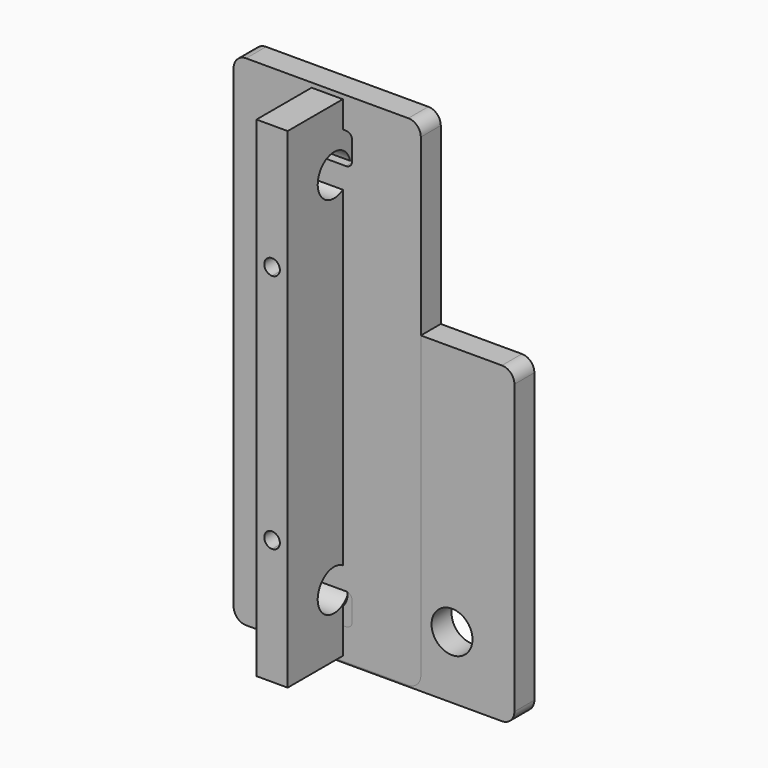
from build123d import *

# Parameters (mm, degrees)
F1_DEPTH  = 5.08
F2_R      = 2.54
F3_R      = 3.571875
F4_DEPTH  = 5.08
F5_R      = 2.54
F6_R      = 1.27
F8_DEPTH  = 19.1135
F9_R      = 4.1656
F10_DEPTH = 25.4


# Not quite as in the source:
# - a feature names something its author has since deleted; it is built from what else it names


with BuildPart() as f1:
    # F0 (on Front) → F1 (new body)
    with BuildSketch(Plane.XZ):
        with BuildLine():
            Line((-4.1654060763, -38.3941942743), (-12.7, -38.3941942743))
            Line((-12.7, -38.3941942743), (-12.7, -51.054))
            Line((-12.7, -51.054), (0, -51.054))
            Line((0, -51.054), (0, -42.5196))
            ThreePointArc((0, -42.5196), (-2.931278739, -41.3137007137), (-4.1654060763, -38.3941942743))
        make_face()
        with BuildLine():
            Line((0, -10.668), (0, -7.9375))
            ThreePointArc((0, -7.9375), (-5.6126600757, -5.6126600757), (-7.9375, 0))
            Line((-7.9375, 0), (-12.7, 0))
            Line((-12.7, 0), (-12.7, -38.3941942743))
            Line((-12.7, -38.3941942743), (-4.1654060763, -38.3941942743))
            ThreePointArc((-4.1654060763, -38.3941942743), (-2.9597007137, -35.422721261), (0, -34.1884))
            Line((0, -34.1884), (0, -10.668))
        make_face()
        with BuildLine():
            ThreePointArc((-7.9375, 0), (-5.6126600757, 5.6126600757), (0, 7.9375))
            Line((0, 7.9375), (0, 12.7))
            Line((0, 12.7), (-12.7, 12.7))
            Line((-12.7, 12.7), (-12.7, 0))
            Line((-12.7, 0), (-7.9375, 0))
        make_face()
        with BuildLine():
            ThreePointArc((0, 7.9375), (5.6126600757, 5.6126600757), (7.9375, 0))
            Line((7.9375, 0), (19.05, 0))
            Line((19.05, 0), (38.1, 0))
            Line((38.1, 0), (38.1, 12.7))
            Line((38.1, 12.7), (0, 12.7))
            Line((0, 12.7), (0, 7.9375))
        make_face()
        with BuildLine():
            Line((38.1, 0), (19.05, 0))
            Line((19.05, 0), (19.05, -38.354))
            Line((19.05, -38.354), (21.2344, -38.354))
            ThreePointArc((21.2344, -38.354), (25.4, -34.1884), (29.5656, -38.354))
            Line((29.5656, -38.354), (38.1, -38.354))
            Line((38.1, -38.354), (38.1, 0))
        make_face()
        with BuildLine():
            Line((21.2344, -38.354), (19.05, -38.354))
            Line((19.05, -38.354), (4.1656, -38.354))
            ThreePointArc((4.1656, -38.354), (2.9455240077, -41.2995240077), (0, -42.5196))
            Line((0, -42.5196), (0, -51.054))
            Line((0, -51.054), (38.1, -51.054))
            Line((38.1, -51.054), (38.1, -38.354))
            Line((38.1, -38.354), (29.5656, -38.354))
            ThreePointArc((29.5656, -38.354), (25.4, -42.5196), (21.2344, -38.354))
        make_face()
        with BuildLine():
            Line((19.05, 0), (7.9375, 0))
            ThreePointArc((7.9375, 0), (5.6126600757, -5.6126600757), (0, -7.9375))
            Line((0, -7.9375), (0, -10.668))
            Line((0, -10.668), (0, -34.1884))
            ThreePointArc((0, -34.1884), (2.9455240077, -35.4084759923), (4.1656, -38.354))
            Line((4.1656, -38.354), (19.05, -38.354))
            Line((19.05, -38.354), (19.05, 0))
        make_face()
    extrude(amount=F1_DEPTH)

    # F2
    f2_edges = [f1.edges().sort_by_distance(p)[0] for p in [
        (38.1, -2.54, 12.7),
        (38.1, -2.54, -51.054),
        (-12.7, -2.54, 12.7),
        (-12.7, -2.54, -51.054),
    ]]
    fillet(f2_edges, radius=F2_R)


with BuildPart() as f4:
    # F3 (on Front) → F4 (new body)
    with BuildSketch(Plane.XZ):
        with BuildLine():
            Line((-8.89, 0), (0, 0))
            Line((0, 0), (0, 16.66875))
            ThreePointArc((0, 16.66875), (-2.38125, 19.05), (0, 21.43125))
            Line((0, 21.43125), (0, 38.1))
            Line((0, 38.1), (-5.08, 38.1))
            Line((-5.08, 38.1), (-5.08, 44.45))
            Line((-5.08, 44.45), (0, 44.45))
            Line((0, 44.45), (0, 50.8))
            Line((0, 50.8), (-19.05, 50.8))
            Line((-19.05, 50.8), (-19.05, 22.225))
            Line((-19.05, 22.225), (-19.05, 0))
            Line((-19.05, 0), (-15.875, 0))
            Line((-15.875, 0), (-8.89, 0))
        make_face()
        with BuildLine():
            ThreePointArc((-6.588125, 22.225), (-10.16, 18.653125), (-13.731875, 22.225))
            ThreePointArc((-13.731875, 22.225), (-10.16, 25.796875), (-6.588125, 22.225))
        make_face(mode=Mode.SUBTRACT)
        Polygon((-15.875, -35.56), (-15.875, 0), (-19.05, 0), (-19.05, -50.8), (0, -50.8), (0, -44.45), (-5.08, -44.45), (-5.08, -38.1), (0, -38.1), (0, -35.56), align=None)
        with BuildLine():
            Line((0, -16.66875), (0, 0))
            Line((0, 0), (-8.89, 0))
            Line((-8.89, 0), (-15.875, 0))
            Line((-15.875, 0), (-15.875, -35.56))
            Line((-15.875, -35.56), (0, -35.56))
            Line((0, -35.56), (0, -21.43125))
            ThreePointArc((0, -21.43125), (-2.38125, -19.05), (0, -16.66875))
        make_face()
        with Locations((-10.16, -22.225)):
            Circle(F3_R, mode=Mode.SUBTRACT)
        with BuildLine():
            Line((0, 16.66875), (0, 0))
            Line((0, 0), (19.05, 0))
            Line((19.05, 0), (19.05, 50.8))
            Line((19.05, 50.8), (0, 50.8))
            Line((0, 50.8), (0, 44.45))
            Line((0, 44.45), (5.08, 44.45))
            Line((5.08, 44.45), (5.08, 38.1))
            Line((5.08, 38.1), (0, 38.1))
            Line((0, 38.1), (0, 21.43125))
            ThreePointArc((0, 21.43125), (1.6837980227, 20.7337980227), (2.38125, 19.05))
            ThreePointArc((2.38125, 19.05), (1.6837980227, 17.3662019773), (0, 16.66875))
        make_face()
        with BuildLine():
            Line((19.05, 0), (0, 0))
            Line((0, 0), (0, -16.66875))
            ThreePointArc((0, -16.66875), (1.6837980227, -17.3662019773), (2.38125, -19.05))
            ThreePointArc((2.38125, -19.05), (1.6837980227, -20.7337980227), (0, -21.43125))
            Line((0, -21.43125), (0, -35.56))
            Line((0, -35.56), (0, -38.1))
            Line((0, -38.1), (5.08, -38.1))
            Line((5.08, -38.1), (5.08, -44.45))
            Line((5.08, -44.45), (0, -44.45))
            Line((0, -44.45), (0, -50.8))
            Line((0, -50.8), (19.05, -50.8))
            Line((19.05, -50.8), (19.05, 0))
        make_face()
    extrude(amount=F4_DEPTH)

    # F5
    f5_edges = [f4.edges().sort_by_distance(p)[0] for p in [
        (19.05, -2.54, 50.8),
        (-19.05, -2.54, 50.8),
        (-19.05, -2.54, -50.8),
        (19.05, -2.54, -50.8),
    ]]
    fillet(f5_edges, radius=F5_R)

    # F6
    f6_edges = [f4.edges().sort_by_distance(p)[0] for p in [
        (5.08, -2.54, 44.45),
        (5.08, -2.54, 38.1),
        (-5.08, -2.54, 44.45),
        (-5.08, -2.54, 38.1),
        (5.08, -2.54, -38.1),
        (-5.08, -2.54, -38.1),
        (5.08, -2.54, -44.45),
        (-5.08, -2.54, -44.45),
    ]]
    fillet(f6_edges, radius=F6_R)


with BuildPart() as f8:
    # F7 (on Front) → F8 (new body)
    with BuildSketch(Plane.XZ):
        with BuildLine():
            Line((0, 22.8854), (0, 0))
            Line((0, 0), (3.175, 0))
            Line((3.175, 0), (3.175, 49.8729))
            Line((3.175, 49.8729), (0, 49.8729))
            Line((0, 49.8729), (0, 26.0604))
            ThreePointArc((0, 26.0604), (1.1225320151, 25.5954320151), (1.5875, 24.4729))
            ThreePointArc((1.5875, 24.4729), (1.1225320151, 23.3503679849), (0, 22.8854))
        make_face()
        with BuildLine():
            Line((-3.175, 0), (0, 0))
            Line((0, 0), (0, 22.8854))
            ThreePointArc((0, 22.8854), (-1.5875, 24.4729), (0, 26.0604))
            Line((0, 26.0604), (0, 49.8729))
            Line((0, 49.8729), (-3.175, 49.8729))
            Line((-3.175, 49.8729), (-3.175, 0))
        make_face()
        with BuildLine():
            Line((0, -22.8854), (0, 0))
            Line((0, 0), (-3.175, 0))
            Line((-3.175, 0), (-3.175, -49.8729))
            Line((-3.175, -49.8729), (0, -49.8729))
            Line((0, -49.8729), (0, -26.0604))
            ThreePointArc((0, -26.0604), (-1.5875, -24.4729), (0, -22.8854))
        make_face()
        with BuildLine():
            Line((3.175, 0), (0, 0))
            Line((0, 0), (0, -22.8854))
            ThreePointArc((0, -22.8854), (1.1225320151, -23.3503679849), (1.5875, -24.4729))
            ThreePointArc((1.5875, -24.4729), (1.1225320151, -25.5954320151), (0, -26.0604))
            Line((0, -26.0604), (0, -49.8729))
            Line((0, -49.8729), (3.175, -49.8729))
            Line((3.175, -49.8729), (3.175, 0))
        make_face()
    extrude(amount=F8_DEPTH)

    # F9 (on face) → F10 (cut)
    with BuildSketch(Plane.YZ.offset(3.175)):
        with Locations((-7.3025, -37.1729)):
            Circle(F9_R)
        with BuildLine():
            ThreePointArc((-3.1369, 37.1729), (-4.3569759923, 40.1184240077), (-7.3025, 41.3385))
            Line((-7.3025, 41.3385), (-7.3025, 37.1729))
            Line((-7.3025, 37.1729), (-3.1369, 37.1729))
        make_face()
        with BuildLine():
            Line((-7.3025, 37.1729), (-7.3025, 41.3385))
            ThreePointArc((-7.3025, 41.3385), (-10.2480240077, 34.2273759923), (-3.1369, 37.1729))
            Line((-3.1369, 37.1729), (-7.3025, 37.1729))
        make_face()
    extrude(amount=-F10_DEPTH, mode=Mode.SUBTRACT)


solid = Compound([f1.part, f4.part, f8.part])
